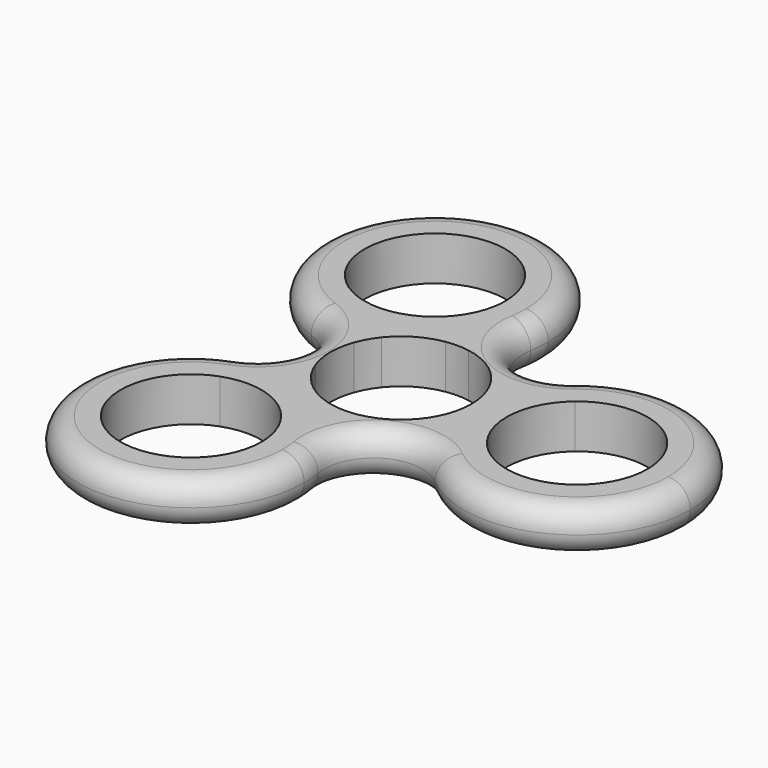
from build123d import *

# Parameters (mm, degrees)
F2_DEPTH = 3.5
F3_R     = 3.49999


# Not quite as in the source:
# - a fillet or chamfer is up to 0.001 mm smaller than in the source, because OpenCascade refuses the exact size
# - a feature names something its author has since deleted; it is built from what else it names


with BuildPart() as f2:
    # F1 (on Top) → F2 (new body, symmetric)
    with BuildSketch(Plane.XY):
        with BuildLine():
            ThreePointArc((46, 0), (35.606388, 16.313885), (16.428571, 13.78775))
            Line((16.428571, 13.78775), (20.8, 8.579044))
            ThreePointArc((20.8, 8.579044), (32.732864, 10.150862), (39.2, 0))
            ThreePointArc((39.2, 0), (32.732864, -10.150862), (20.8, -8.579044))
            Line((20.8, -8.579044), (16.428571, -13.78775))
            ThreePointArc((16.428571, -13.78775), (35.606388, -16.313885), (46, 0))
        make_face()
        with BuildLine():
            Line((-2.97033, 22.302851), (3.726256, 21.121435))
            ThreePointArc((3.726256, 21.121435), (3.931433, 22.679094), (4, 24.248711))
            ThreePointArc((4, 24.248711), (-24.325045, 38.99298), (-20.154827, 7.333685))
            Line((-20.154827, 7.333685), (-17.82967, 13.723806))
            ThreePointArc((-17.82967, 13.723806), (-20.424472, 33.422923), (-2.8, 24.248711))
            ThreePointArc((-2.8, 24.248711), (-2.842664, 23.272061), (-2.97033, 22.302851))
        make_face()
        with BuildLine():
            ThreePointArc((4, -24.248711), (3.931433, -22.679094), (3.726256, -21.121435))
            Line((3.726256, -21.121435), (-2.97033, -22.302851))
            ThreePointArc((-2.97033, -22.302851), (-2.842664, -23.272061), (-2.8, -24.248711))
            ThreePointArc((-2.8, -24.248711), (-20.424472, -33.422923), (-17.82967, -13.723806))
            Line((-17.82967, -13.723806), (-20.154827, -7.333685))
            ThreePointArc((-20.154827, -7.333685), (-24.325045, -38.99298), (4, -24.248711))
        make_face()
        with BuildLine():
            ThreePointArc((1.945861, 11.02967), (5.6, 9.699485), (8.579044, 7.2))
            Line((8.579044, 7.2), (16.428571, 13.78775))
            ThreePointArc((16.428571, 13.78775), (7.509615, 13.007034), (3.726256, 21.121435))
            Line((3.726256, 21.121435), (1.945861, 11.02967))
        make_face()
        with BuildLine():
            ThreePointArc((-10.524905, -3.82967), (-11.2, 0), (-10.524905, 3.82967))
            Line((-10.524905, 3.82967), (-20.154827, 7.333685))
            ThreePointArc((-20.154827, 7.333685), (-15.019229, 0), (-20.154827, -7.333685))
            Line((-20.154827, -7.333685), (-10.524905, -3.82967))
        make_face()
        with BuildLine():
            Line((16.428571, -13.78775), (8.579044, -7.2))
            ThreePointArc((8.579044, -7.2), (5.6, -9.699485), (1.945861, -11.02967))
            Line((1.945861, -11.02967), (3.726256, -21.121435))
            ThreePointArc((3.726256, -21.121435), (7.509615, -13.007034), (16.428571, -13.78775))
        make_face()
        with BuildLine():
            ThreePointArc((-1.747066, 11.0629), (1.810803, 15.64531), (3.726256, 21.121435))
            Line((3.726256, 21.121435), (-2.97033, 22.302851))
            ThreePointArc((-2.97033, 22.302851), (-8.4, 14.549227), (-17.82967, 13.723806))
            Line((-17.82967, 13.723806), (-20.154827, 7.333685))
            ThreePointArc((-20.154827, 7.333685), (-14.454637, 6.254454), (-8.707219, 7.044454))
            ThreePointArc((-8.707219, 7.044454), (-5.6, 9.699485), (-1.747066, 11.0629))
        make_face()
        with BuildLine():
            Line((-20.154827, 7.333685), (-10.524905, 3.82967))
            ThreePointArc((-10.524905, 3.82967), (-9.74948, 5.512498), (-8.707219, 7.044454))
            ThreePointArc((-8.707219, 7.044454), (-14.454637, 6.254454), (-20.154827, 7.333685))
        make_face()
        with BuildLine():
            ThreePointArc((-1.747066, 11.0629), (0.100776, 11.199547), (1.945861, 11.02967))
            Line((1.945861, 11.02967), (3.726256, 21.121435))
            ThreePointArc((3.726256, 21.121435), (1.810803, 15.64531), (-1.747066, 11.0629))
        make_face()
        with BuildLine():
            ThreePointArc((-8.707219, -7.044454), (-9.74948, -5.512498), (-10.524905, -3.82967))
            Line((-10.524905, -3.82967), (-20.154827, -7.333685))
            ThreePointArc((-20.154827, -7.333685), (-14.454637, -6.254454), (-8.707219, -7.044454))
        make_face()
        with BuildLine():
            Line((-2.97033, -22.302851), (3.726256, -21.121435))
            ThreePointArc((3.726256, -21.121435), (1.810803, -15.64531), (-1.747066, -11.0629))
            ThreePointArc((-1.747066, -11.0629), (-5.6, -9.699485), (-8.707219, -7.044454))
            ThreePointArc((-8.707219, -7.044454), (-14.454637, -6.254454), (-20.154827, -7.333685))
            Line((-20.154827, -7.333685), (-17.82967, -13.723806))
            ThreePointArc((-17.82967, -13.723806), (-8.4, -14.549227), (-2.97033, -22.302851))
        make_face()
        with BuildLine():
            Line((3.726256, -21.121435), (1.945861, -11.02967))
            ThreePointArc((1.945861, -11.02967), (0.100776, -11.199547), (-1.747066, -11.0629))
            ThreePointArc((-1.747066, -11.0629), (1.810803, -15.64531), (3.726256, -21.121435))
        make_face()
        with BuildLine():
            ThreePointArc((8.579044, 7.2), (9.648704, 5.687048), (10.454286, 4.018446))
            ThreePointArc((10.454286, 4.018446), (12.643834, 9.390856), (16.428571, 13.78775))
            Line((16.428571, 13.78775), (8.579044, 7.2))
        make_face()
        with BuildLine():
            ThreePointArc((10.454286, 4.018446), (11.011993, 2.043526), (11.2, 0))
            ThreePointArc((11.2, 0), (11.011993, -2.043526), (10.454286, -4.018446))
            ThreePointArc((10.454286, -4.018446), (12.643834, -9.390856), (16.428571, -13.78775))
            Line((16.428571, -13.78775), (20.8, -8.579044))
            ThreePointArc((20.8, -8.579044), (16.8, 0), (20.8, 8.579044))
            Line((20.8, 8.579044), (16.428571, 13.78775))
            ThreePointArc((16.428571, 13.78775), (12.643834, 9.390856), (10.454286, 4.018446))
        make_face()
        with BuildLine():
            ThreePointArc((16.428571, -13.78775), (12.643834, -9.390856), (10.454286, -4.018446))
            ThreePointArc((10.454286, -4.018446), (9.648704, -5.687048), (8.579044, -7.2))
            Line((8.579044, -7.2), (16.428571, -13.78775))
        make_face()
    extrude(amount=F2_DEPTH, both=True)

    # F3 (radius 3.5 in the source; OpenCascade refuses exactly that, so slightly less here)
    f3_edges = [f2.edges().sort_by_distance(p)[0] for p in [
        (-23, -39.837169, 3.5),
        (-23, 39.837169, 3.5),
        (46, 0, 3.5),
        (-23, -39.837169, -3.5),
        (46, 0, -3.5),
        (-23, 39.837169, -3.5),
    ]]
    fillet(f3_edges, radius=F3_R)


solid = f2.part
